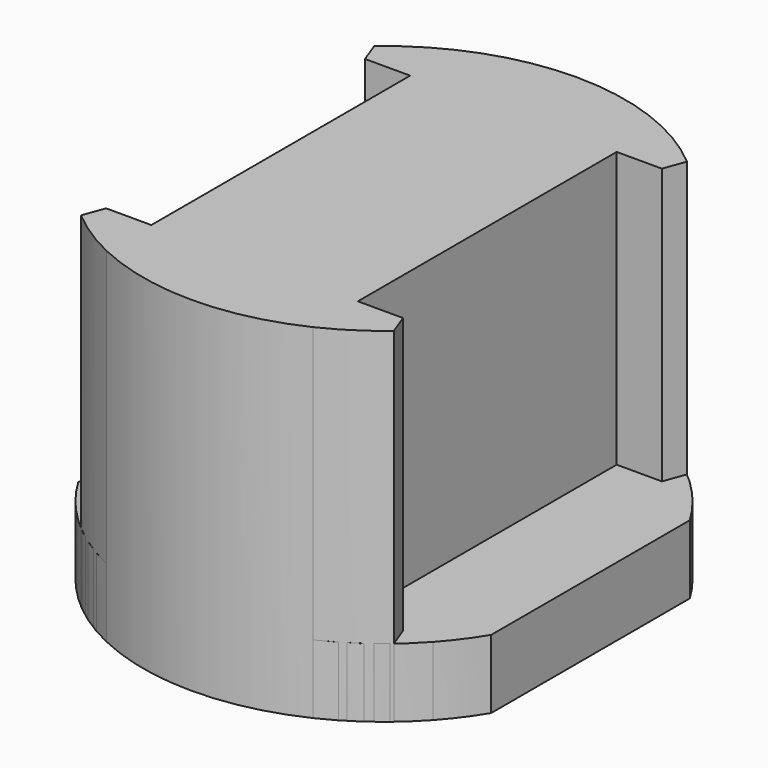
from build123d import *

# Parameters (mm, degrees)
F1_DEPTH    = 5
F0_W        = 15
F0_H        = 23.5
F0_W_2      = 6.2
F0_H_2      = 13
F2_DEPTH    = 25
F3_DEPTH    = 15.6
F4_T1_DEPTH = 36.3750267574


# Not quite as in the source:
# - a fillet or chamfer that OpenCascade refuses, or shapes differently, is made with other operations: its cross-section is extruded or revolved along the edge and cut away or added
# - a feature names something its author has since deleted; it is built from what else it names


with BuildPart() as f1:
    # F0 (on Top) → F1 (new body)
    with BuildSketch(Plane.XY):
        with BuildLine():
            Line((15, -9.0138781887), (15, 9.0138781887))
            ThreePointArc((15, 9.0138781887), (14.0511141288, 10.4314999755), (12.9687123493, 11.75))
            Line((12.9687123493, 11.75), (7.5, 11.75))
            Line((7.5, 11.75), (7.5, -11.75))
            Line((7.5, -11.75), (12.9687123493, -11.75))
            ThreePointArc((12.9687123493, -11.75), (14.0511141288, -10.4314999755), (15, -9.0138781887))
        make_face()
        with BuildLine():
            ThreePointArc((7.5, -15.8113883008), (10.4338758399, -14.0493499834), (12.9687123493, -11.75))
            Line((12.9687123493, -11.75), (7.5, -11.75))
            Line((7.5, -11.75), (7.5, -15.8113883008))
        make_face()
        with BuildLine():
            Line((7.5, 11.75), (12.9687123493, 11.75))
            ThreePointArc((12.9687123493, 11.75), (10.4338758399, 14.0493499834), (7.5, 15.8113883008))
            Line((7.5, 15.8113883008), (7.5, 11.75))
        make_face()
    extrude(amount=F1_DEPTH)


with BuildPart() as f1b:
    # F0 (on Top) → F1, piece 2 (new body)
    with BuildSketch(Plane.XY):
        with BuildLine():
            Line((-7.5, -11.75), (-7.5, 11.75))
            Line((-7.5, 11.75), (-12.9687123493, 11.75))
            ThreePointArc((-12.9687123493, 11.75), (-14.0511141288, 10.4314999755), (-15, 9.0138781887))
            Line((-15, 9.0138781887), (-15, -9.0138781887))
            ThreePointArc((-15, -9.0138781887), (-14.0511141288, -10.4314999755), (-12.9687123493, -11.75))
            Line((-12.9687123493, -11.75), (-7.5, -11.75))
        make_face()
        with BuildLine():
            Line((-7.5, 11.75), (-7.5, 15.8113883008))
            ThreePointArc((-7.5, 15.8113883008), (-10.4338758399, 14.0493499834), (-12.9687123493, 11.75))
            Line((-12.9687123493, 11.75), (-7.5, 11.75))
        make_face()
        with BuildLine():
            ThreePointArc((-12.9687123493, -11.75), (-10.4338758399, -14.0493499834), (-7.5, -15.8113883008))
            Line((-7.5, -15.8113883008), (-7.5, -11.75))
            Line((-7.5, -11.75), (-12.9687123493, -11.75))
        make_face()
    extrude(amount=F1_DEPTH)


with BuildPart() as f2:
    # F0 (on Top) → F2 (new body)
    with BuildSketch(Plane.XY):
        Rectangle(F0_W, F0_H)
        Rectangle(F0_W_2, F0_H_2, mode=Mode.SUBTRACT)
        Rectangle(F0_W_2, F0_H_2)
        with BuildLine():
            Line((7.5, 11.75), (7.5, 15.8113883008))
            ThreePointArc((7.5, 15.8113883008), (0, 17.5), (-7.5, 15.8113883008))
            Line((-7.5, 15.8113883008), (-7.5, 11.75))
            Line((-7.5, 11.75), (7.5, 11.75))
        make_face()
        with BuildLine():
            ThreePointArc((-7.5, -15.8113883008), (0, -17.5), (7.5, -15.8113883008))
            Line((7.5, -15.8113883008), (7.5, -11.75))
            Line((7.5, -11.75), (-7.5, -11.75))
            Line((-7.5, -11.75), (-7.5, -15.8113883008))
        make_face()
        with BuildLine():
            ThreePointArc((-12.9687123493, -11.75), (-10.4338758399, -14.0493499834), (-7.5, -15.8113883008))
            Line((-7.5, -15.8113883008), (-7.5, -11.75))
            Line((-7.5, -11.75), (-12.9687123493, -11.75))
        make_face()
        with BuildLine():
            Line((-7.5, 11.75), (-7.5, 15.8113883008))
            ThreePointArc((-7.5, 15.8113883008), (-10.4338758399, 14.0493499834), (-12.9687123493, 11.75))
            Line((-12.9687123493, 11.75), (-7.5, 11.75))
        make_face()
        with BuildLine():
            Line((7.5, 11.75), (12.9687123493, 11.75))
            ThreePointArc((12.9687123493, 11.75), (10.4338758399, 14.0493499834), (7.5, 15.8113883008))
            Line((7.5, 15.8113883008), (7.5, 11.75))
        make_face()
        with BuildLine():
            ThreePointArc((7.5, -15.8113883008), (10.4338758399, -14.0493499834), (12.9687123493, -11.75))
            Line((12.9687123493, -11.75), (7.5, -11.75))
            Line((7.5, -11.75), (7.5, -15.8113883008))
        make_face()
    extrude(amount=F2_DEPTH)

    # F0 (on Top) → F3 (cut)
    with BuildSketch(Plane.XY):
        Rectangle(F0_W_2, F0_H_2)
    extrude(amount=F3_DEPTH, mode=Mode.SUBTRACT)

    # F4: chamfer of 2 on 4 edges, made by hand

    # F4_s2 → F4_t1 (cut)
    with BuildSketch(Plane.XY.offset(-5.6875133787)):
        with BuildLine():
            Line((-11.3881617362, -13.3863096005), (-10.7571586121, -11.6749396443))
            Line((-10.7571586121, -11.6749396443), (-10.7571586121, -11.6349396443))
            ThreePointArc((-10.7571586121, -11.6349396443), (-11.8629354807, -11.71), (-12.9687123493, -11.71))
            Line((-12.9687123493, -11.71), (-12.9983551204, -11.7768571429))
            ThreePointArc((-12.9983551204, -11.7768571429), (-12.2058182488, -12.5964122224), (-11.4141285615, -13.4167353131))
            Line((-11.4141285615, -13.4167353131), (-11.3881617362, -13.3863096005))
        make_face()
        with BuildLine():
            Line((10.7571586121, -11.6749396443), (11.3881617362, -13.3863096005))
            Line((11.3881617362, -13.3863096005), (11.4141285615, -13.4167353131))
            ThreePointArc((11.4141285615, -13.4167353131), (12.2058182488, -12.5964122224), (12.9983551204, -11.7768571429))
            Line((12.9983551204, -11.7768571429), (12.9687123493, -11.71))
            ThreePointArc((12.9687123493, -11.71), (11.8629354807, -11.71), (10.7571586121, -11.6349396443))
            Line((10.7571586121, -11.6349396443), (10.7571586121, -11.6749396443))
        make_face()
        with BuildLine():
            Line((10.7571586121, 11.6749396443), (11.3881617362, 13.3863096005))
            Line((11.3881617362, 13.3863096005), (11.4141285615, 13.4167353131))
            ThreePointArc((11.4141285615, 13.4167353131), (12.2058182488, 12.5964122224), (12.9983551204, 11.7768571429))
            Line((12.9983551204, 11.7768571429), (12.9687123493, 11.71))
            ThreePointArc((12.9687123493, 11.71), (11.8629354807, 11.71), (10.7571586121, 11.6349396443))
            Line((10.7571586121, 11.6349396443), (10.7571586121, 11.6749396443))
        make_face()
        with BuildLine():
            Line((-11.3881617362, 13.3863096005), (-10.7571586121, 11.6749396443))
            Line((-10.7571586121, 11.6749396443), (-10.7571586121, 11.6349396443))
            ThreePointArc((-10.7571586121, 11.6349396443), (-11.8629354807, 11.71), (-12.9687123493, 11.71))
            Line((-12.9687123493, 11.71), (-12.9983551204, 11.7768571429))
            ThreePointArc((-12.9983551204, 11.7768571429), (-12.2058182488, 12.5964122224), (-11.4141285615, 13.4167353131))
            Line((-11.4141285615, 13.4167353131), (-11.3881617362, 13.3863096005))
        make_face()
    extrude(amount=F4_T1_DEPTH, mode=Mode.SUBTRACT)


solid = Compound([f1.part, f1b.part, f2.part])
